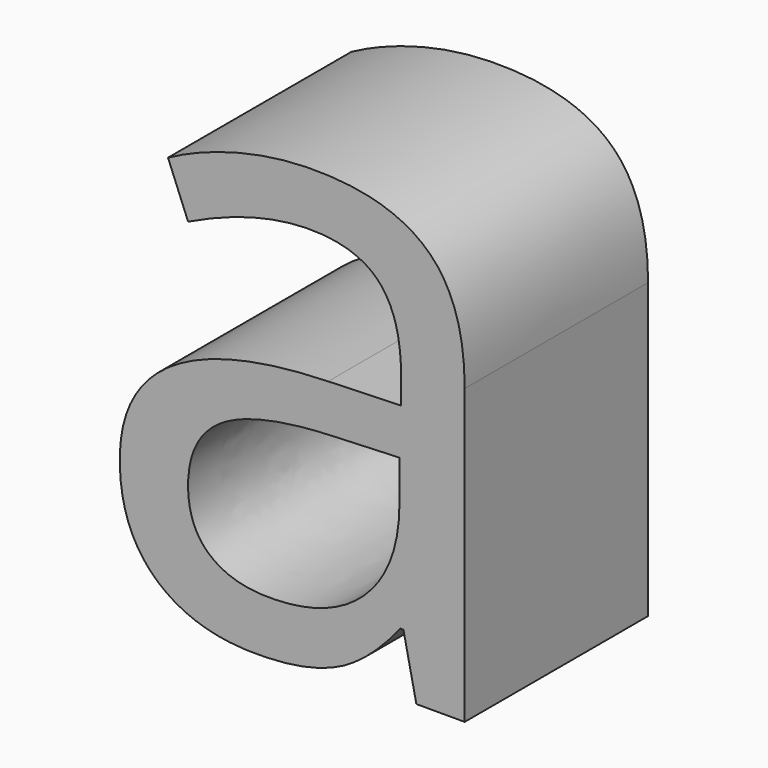
from build123d import *

# Parameters (mm, degrees)
F0_TEXT_SIZE = 44.515904867
F1_DEPTH     = 12.7


# Not quite as in the source:
# - Text() gives the source's letters only with a copy of the font that has no kerning and outlines rounded to 1/6400 em; it was checked with that copy


with BuildPart() as f1:
    # F0 (on Front) → F1 (new body)
    with BuildSketch(Plane.XZ):
        with Locations((-58.5436783731, 0)):
            Text('a', F0_TEXT_SIZE, font='Open Sans', text_align=(TextAlign.LEFT, TextAlign.BOTTOM))
    extrude(amount=F1_DEPTH)


solid = f1.part
